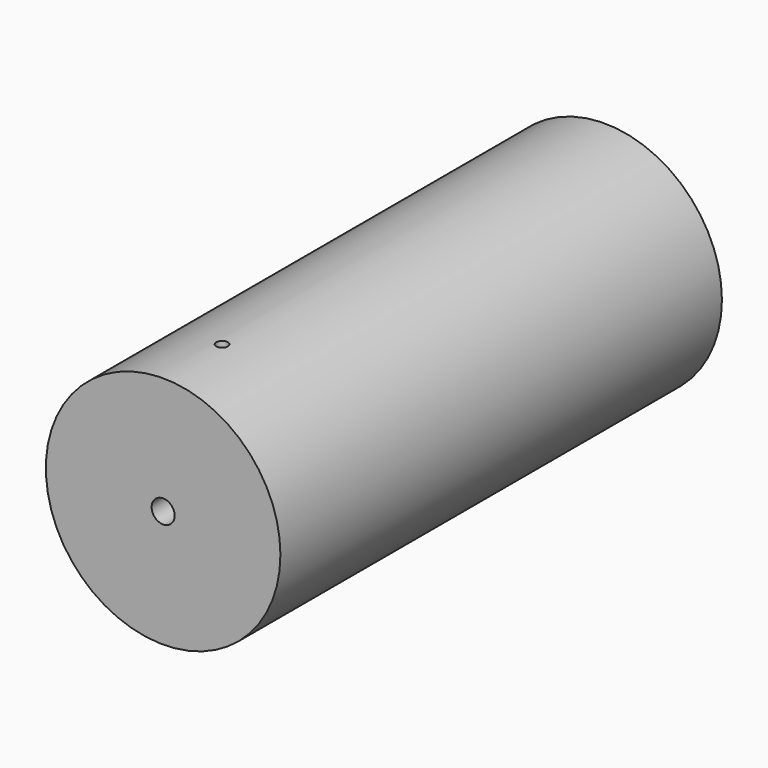
from build123d import *

# Parameters (mm, degrees)
F0_R     = 25.5
F0_R_2   = 2.5
F1_DEPTH = 120
F3_D     = 2.5
F3_DEPTH = 25.501


# Not quite as in the source:
# - a feature names something its author has since deleted; it is built from what else it names


with BuildPart() as f1:
    # F0 (on Front) → F1 (new body)
    with BuildSketch(Plane.XZ):
        Circle(F0_R)
        Circle(F0_R_2, mode=Mode.SUBTRACT)
    extrude(amount=F1_DEPTH)

    # F3 (through all, one way)
    with BuildSketch(Plane(origin=(0, 0, 0), x_dir=(1, 0, 0), z_dir=(0, 0, -1))):
        with Locations((0, 104)):
            Circle(F3_D / 2)
    extrude(amount=-F3_DEPTH, mode=Mode.SUBTRACT)


solid = f1.part
